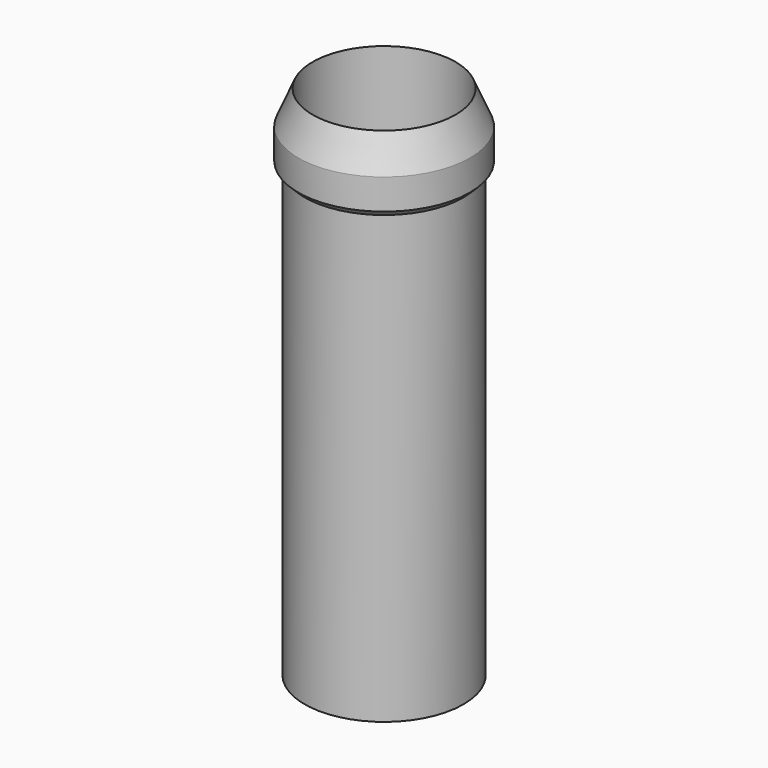
from build123d import *

# Parameters (mm, degrees)
F0_R        = 15.875
F0_R_2      = 14.2875
F1_DEPTH    = 44.45
F2_R        = 17.145
F2_R_2      = 14.2875
F3_DEPTH    = 16.51
F5_S5_R     = 15.875
F5_T6_DEPTH = 26


# Not quite as in the source:
# - a fillet or chamfer that OpenCascade refuses, or shapes differently, is made with other operations: its cross-section is extruded or revolved along the edge and cut away or added


with BuildPart() as f1:
    # F0 (on Top) → F1 (new body, symmetric)
    with BuildSketch(Plane.XY):
        Circle(F0_R)
        Circle(F0_R_2, mode=Mode.SUBTRACT)
    extrude(amount=F1_DEPTH, both=True)

    # F2 (on face) → F3 (join)
    with BuildSketch(Plane.XY.offset(44.45)):
        Circle(F2_R)
        Circle(F2_R_2, mode=Mode.SUBTRACT)
    extrude(amount=F3_DEPTH)

    # F4: chamfer of 3.81 x 8.89 on 1 edges, made by hand

    # F4_s1 → F4_t2 (revolve, cut)
    with BuildSketch(Plane.XZ):
        Polygon((17.145, 52.07), (13.335, 60.96), (17.145, 60.96), align=None)
    revolve(axis=Axis((0, 0, 60.96), (0, 0, 1)), mode=Mode.SUBTRACT)

    # F5: chamfer of 1.524 on 1 edges, made by hand


with BuildPart() as f5_tool2:
    # F5_s3 → F5_t4 (revolve)
    with BuildSketch(Plane.XZ):
        Polygon((15.621, 44.45), (17.145, 45.974), (17.145, 44.45), align=None)
    revolve(axis=Axis((0, 0, 44.45), (0, 0, 1)))

    # F5_s5 → F5_t6 (cut, symmetric)
    with BuildSketch(Plane.XY.offset(45.2)):
        Circle(F5_S5_R)
    extrude(amount=F5_T6_DEPTH, both=True, mode=Mode.SUBTRACT)


with BuildPart() as f1_1:
    add(f1.part)

    # F5_t1: cut F5_tool2
    add(f5_tool2.part, mode=Mode.SUBTRACT)


solid = f1_1.part
